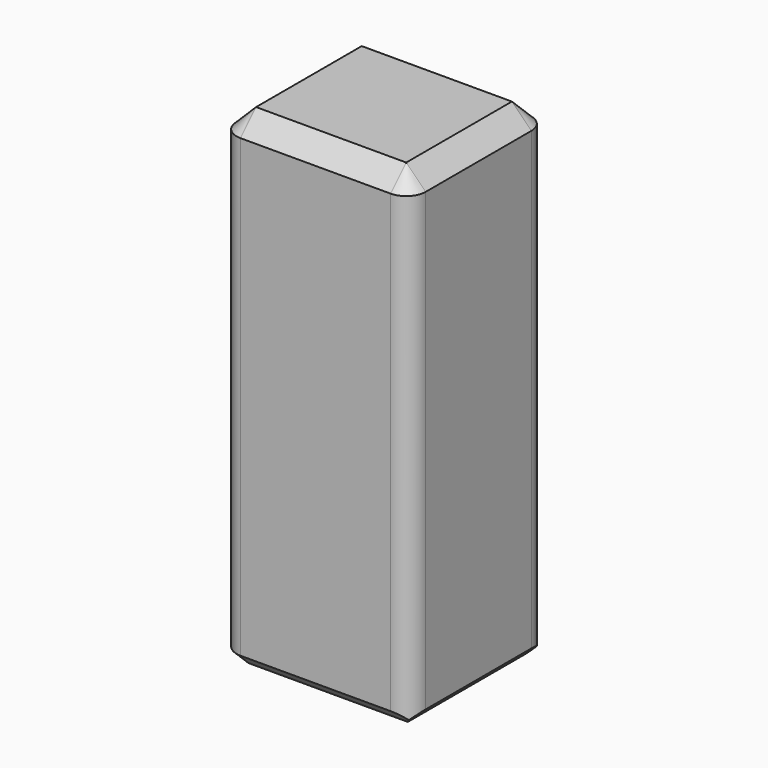
from build123d import *

# Parameters (mm, degrees)
F0_W         = 48.5600655451
F0_H         = 43.9142854884
F0_W_2       = 42.5600655451
F0_H_2       = 37.9142854884
F1_DEPTH     = 127
F2_DEPTH     = 3
F3_R         = 5
F4_T1_DEPTH  = 51.7727004283
F4_T3_DEPTH  = 69.6311153681
F4_T5_DEPTH  = 74.2768954248
F4_T7_DEPTH  = 56.418480485
F4_T10_ANGLE = 90
F5_R         = 5
F6_SIZE      = 5


# Not quite as in the source:
# - a fillet or chamfer that OpenCascade refuses, or shapes differently, is made with other operations: its cross-section is extruded or revolved along the edge and cut away or added


with BuildPart() as f1:
    # F0 (on Top) → F1 (new body)
    with BuildSketch(Plane.XY):
        with Locations((13.9204316549, -10.4247569107)):
            Rectangle(F0_W, F0_H)
        with Locations((13.9204316549, -10.4247569107)):
            Rectangle(F0_W_2, F0_H_2, mode=Mode.SUBTRACT)
    extrude(amount=-F1_DEPTH)

    # F0 (on Top) → F2 (join)
    with BuildSketch(Plane.XY):
        with Locations((13.9204316549, -10.4247569107)):
            Rectangle(F0_W_2, F0_H_2)
    extrude(amount=-F2_DEPTH)

    # F3
    f3_edges = [f1.edges().sort_by_distance(p)[0] for p in [
        (-10.359601, -32.3819, -63.5),
    ]]
    fillet(f3_edges, radius=F3_R)

    # F4: chamfer of 5 on 3 edges, made by hand

    # F4_s2 → F4_t1 (cut)
    with BuildSketch(Plane.XZ.offset(-24.3908007734)):
        Polygon((-10.3596011177, -122), (-5.3596011177, -127), (-10.3596011177, -127), align=None)
    extrude(amount=F4_T1_DEPTH, mode=Mode.SUBTRACT)

    # F4_s4 → F4_t3 (cut)
    with BuildSketch(Plane.XZ.offset(-24.3908007734)):
        Polygon((33.2004644275, -127), (38.2004644275, -122), (38.2004644275, -127), align=None)
    extrude(amount=F4_T3_DEPTH, mode=Mode.SUBTRACT)

    # F4_s6 → F4_t5 (cut)
    with BuildSketch(Plane.YZ.offset(-23.2180160575)):
        Polygon((11.5323858336, -122), (6.5323858336, -127), (11.5323858336, -127), align=None)
    extrude(amount=F4_T5_DEPTH, mode=Mode.SUBTRACT)

    # F4_s8 → F4_t7 (cut)
    with BuildSketch(Plane.YZ.offset(-5.3596011177)):
        Polygon((-27.3818996549, -127), (-32.3818996549, -122), (-32.3818996549, -127), align=None)
    extrude(amount=F4_T7_DEPTH, mode=Mode.SUBTRACT)

    # F4_s9 → F4_t10 (revolve, cut)
    with BuildSketch(Plane.XZ.offset(27.3818996549)):
        Polygon((-10.3596011177, -122), (-5.3596011177, -127), (-10.3596011177, -127), align=None)
    revolve(axis=Axis((-5.3596011177, -27.3818996549, -127), (0, 0, 1)), revolution_arc=F4_T10_ANGLE, mode=Mode.SUBTRACT)

    # F5
    f5_edges = [f1.edges().sort_by_distance(p)[0] for p in [
        (-10.359601, 11.532386, -61),
        (38.200464, 11.532386, -61),
        (38.200464, -32.3819, -61),
    ]]
    fillet(f5_edges, radius=F5_R)

    # F6
    f6_edges = [f1.edges().sort_by_distance(p)[0] for p in [
        (13.920432, -32.3819, 0),
    ]]
    chamfer(f6_edges, length=F6_SIZE)


solid = f1.part
